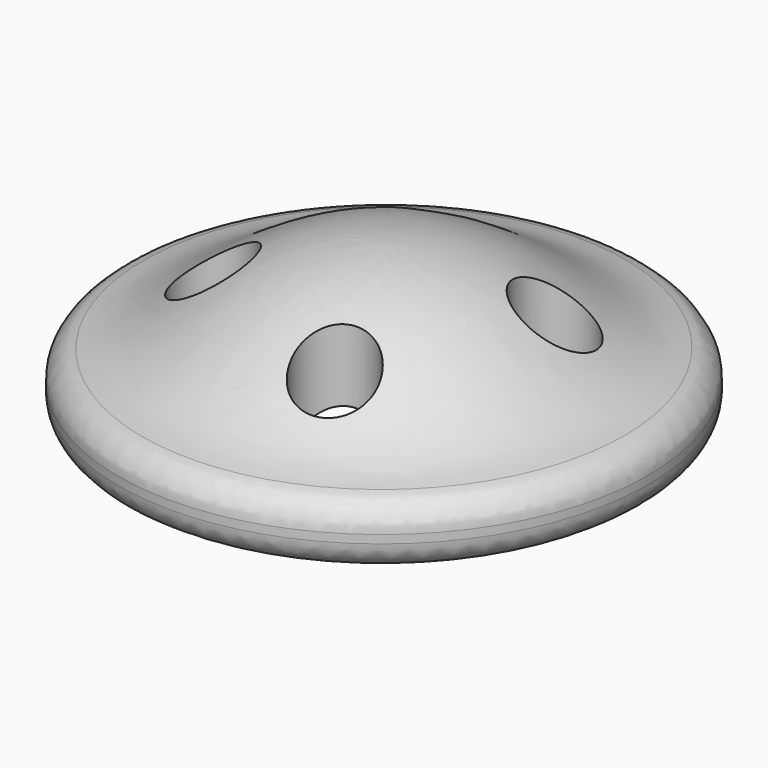
from build123d import *

# Parameters (mm, degrees)
F2_R     = 17.1907282967
F3_DEPTH = 62.6266673207
F4_R     = 12.7
F6_ANGLE = -180


with BuildPart() as f1:
    # F0 (on Front) → F1 (revolve)
    with BuildSketch(Plane.XZ):
        with BuildLine():
            add(Edge.make_bspline(
                [(-152.812341915, 0), (-100.8551691969, -0.2522269885), (-88.6408338944, 43.1802446644), (-31.6110518421, 43.0588798813)],
                knots=[0, 0, 0, 0, 128.6227812324, 128.6227812324, 128.6227812324, 128.6227812324], degree=3))
            Line((-152.812341915, 0), (-152.9538370747, -29.1471126777))
            add(Edge.make_bspline(
                [(-152.9538370747, -29.1471126777), (-148.6899477355, -29.1678118018), (-140.4014386252, -28.760155914), (-128.7575491359, -26.8944523918), (-118.013724725, -23.9536032729), (-108.2543438045, -20.2038308388), (-99.4870098016, -15.9539060142), (-91.6378234912, -11.4997861798), (-84.5808573048, -7.0897753947), (-78.1731425852, -2.91515259), (-72.2769679376, 0.8867042748), (-66.7648015414, 4.2284417428), (-61.5080430699, 7.0709774217), (-56.3534957324, 9.4182026316), (-51.0972213662, 11.2984999455), (-45.4731209064, 12.7292769237), (-39.1714456936, 13.6771880547), (-34.3119784708, 13.917105587), (-31.6730802517, 13.9114897614)],
                knots=[0, 0, 0, 0, 0.0625, 0.125, 0.1875, 0.25, 0.3125, 0.375, 0.4375, 0.5, 0.5625, 0.625, 0.6875, 0.75, 0.8125, 0.875, 0.9375, 1, 1, 1, 1], degree=3))
            Line((-31.6730802517, 13.9114897614), (-31.6110518421, 43.0588798813))
        make_face()
    revolve(axis=Axis((-152.8830894949, 0, -14.5735563388), (-0.00485446, 0, -0.999988217)))

    # F2 (on Top) → F3 (cut, symmetric)
    with BuildSketch(Plane.XY):
        with Locations((-128.2407670775, 58.7333589792)):
            Circle(F2_R)
        with Locations((-94.0085962196, -24.5011881213)):
            Circle(F2_R)
        with Locations((-177.2431433201, -58.7333589792)):
            Circle(F2_R)
        with Locations((-211.475314178, 24.5011881213)):
            Circle(F2_R)
    extrude(amount=F3_DEPTH, both=True, mode=Mode.SUBTRACT)

    # F4
    f4_edges = [f1.edges().sort_by_distance(p)[0] for p in [
        (-273.81083, 0, 15.086952),
        (-273.589869, 0, 44.23357),
    ]]
    fillet(f4_edges, radius=F4_R)


with BuildPart() as f1_1:
    # F6: moved
    add(f1.part.rotate(Axis((96.6221243143, 0, 11.4439129829), (1, 0, 0)), F6_ANGLE))


solid = f1_1.part
